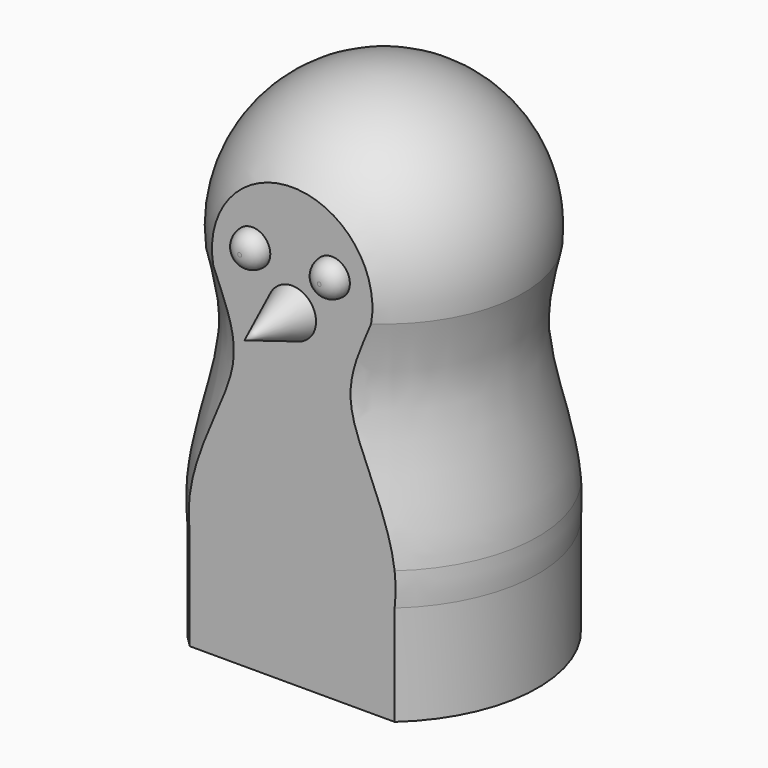
from build123d import *

# Parameters (mm, degrees)
F3_DEPTH      = 177.8
F3_DEPTH_BACK = 12.7
F4_R          = 7.62
F5_DEPTH      = 19.05
F6_SIZE2      = 18.860161823
F6_SIZE       = 7.62
F4_R_2        = 5.715
F7_DEPTH      = 5.08
F8_R          = 5.07999
F9_R          = 6.139399456
F10_DEPTH     = 50.8
F11_SCALE     = 0.51715159


# Not quite as in the source:
# - a fillet or chamfer is up to 0.001 mm smaller than in the source, because OpenCascade refuses the exact size


with BuildPart() as f1:
    # F0 (on Front) → F1 (revolve)
    with BuildSketch(Plane.XZ):
        with BuildLine():
            Line((-6.139399456, 0), (0, 0))
            Line((0, 0), (0, 146.0500033258))
            Line((0, 146.0500033258), (0, 152.4))
            ThreePointArc((0, 152.4), (-33.2006597867, 137.6319951518), (-44.4655865431, 103.0852268133))
            add(Edge.make_bspline(
                [(-49.1152013464, 36.1084283333), (-48.0326439436, 49.6014705241), (-37.8272166921, 76.0482431769), (-42.543614325, 94.8604386904), (-44.4655865431, 103.0852268133)],
                knots=[0.3424224234, 0.3424224234, 0.3424224234, 0.3424224234, 0.7066775859, 1, 1, 1, 1], degree=3))
            Line((-49.1152013464, 36.1084283333), (-49.1152013464, 25.6455829718))
            add(Edge.make_bspline(
                [(-44.4655865431, 0), (-46.3688797408, 8.4610342592), (-48.4665187415, 16.8703142107), (-49.1152013464, 25.6455829718)],
                knots=[0, 0, 0, 0, 0.246321171, 0.246321171, 0.246321171, 0.246321171], degree=3))
            Line((-44.4655865431, 0), (-38.2711647941, 0))
            Line((-38.2711647941, 0), (-6.139399456, 0))
        make_face()
        Polygon((-6.139399456, -6.35), (-6.139399456, 0), (-38.2711647941, 0), (-44.4655865431, 0), (-44.4655865431, -6.35), align=None)
        with BuildLine():
            Line((-44.4655865431, -6.35), (-44.4655865431, 0))
            add(Edge.make_bspline(
                [(-44.4655865431, 0), (-46.3688797408, 8.4610342592), (-48.4665187415, 16.8703142107), (-49.1152013464, 25.6455829718)],
                knots=[0, 0, 0, 0, 0.246321171, 0.246321171, 0.246321171, 0.246321171], degree=3))
            Line((-49.1152013464, 25.6455829718), (-49.1152013464, 0))
            Line((-49.1152013464, 0), (-49.1152013464, -6.35))
            Line((-49.1152013464, -6.35), (-44.4655865431, -6.35))
        make_face()
        with BuildLine():
            add(Edge.make_bspline(
                [(-49.1152013464, 25.6455829718), (-49.3682823563, 29.0692201465), (-49.4008119098, 32.5485659437), (-49.1152013464, 36.1084283333)],
                knots=[0.246321171, 0.246321171, 0.246321171, 0.246321171, 0.3424224234, 0.3424224234, 0.3424224234, 0.3424224234], degree=3))
            Line((-49.1152013464, 25.6455829718), (-49.1152013464, 36.1084283333))
        make_face()
    revolve(axis=Axis((0, 0, 76.2), (0, 0, 1)))

    # F2 (on Top) → F3 (cut, two sides)
    with BuildSketch(Plane.XY) as f3_sk:
        Polygon((25.6092443837, -36.641700535), (-25.1907556163, -36.641700535), (-46.7807556163, -36.641700535), (-46.7807556163, -67.121700535), (42.1192443837, -67.121700535), (42.1192443837, -36.641700535), align=None)
    extrude(amount=F3_DEPTH, mode=Mode.SUBTRACT)
    extrude(f3_sk.sketch, amount=-F3_DEPTH_BACK, mode=Mode.SUBTRACT)

    # F4 (on face) → F5 (join)
    with BuildSketch(Plane.XZ.offset(36.641700535)):
        with Locations((0, 97.9992443837)):
            Circle(F4_R)
    extrude(amount=F5_DEPTH)

    # F6
    f6_edges = [f1.edges().sort_by_distance(p)[0] for p in [
        (-7.62, -55.691701, 97.999244),
    ]]
    f6_side = f1.faces().sort_by_distance((0, -55.691701, 97.999244))[0]
    chamfer(f6_edges, length=F6_SIZE, length2=F6_SIZE2, reference=f6_side)

    # F4 (on face) → F7 (join)
    with BuildSketch(Plane.XZ.offset(36.641700535)):
        with Locations((-12.7, 112.2232443837)):
            Circle(F4_R_2)
        with Locations((12.7, 112.2232443837)):
            Circle(F4_R_2)
    extrude(amount=F7_DEPTH)

    # F8 (radius 5.08 in the source; OpenCascade refuses exactly that, so slightly less here)
    f8_edges = [f1.edges().sort_by_distance(p)[0] for p in [
        (-18.415, -41.721701, 112.223244),
        (6.985, -41.721701, 112.223244),
    ]]
    fillet(f8_edges, radius=F8_R)

    # F9 (on face) → F10 (cut)
    with BuildSketch(Plane(origin=(0, 0, -6.35), x_dir=(1, 0, 0), z_dir=(0, 0, -1))):
        Circle(F9_R)
    extrude(amount=-F10_DEPTH, mode=Mode.SUBTRACT)


with BuildPart() as f1_1:
    # F11: moved
    add(f1.part.scale(F11_SCALE))


solid = f1_1.part
